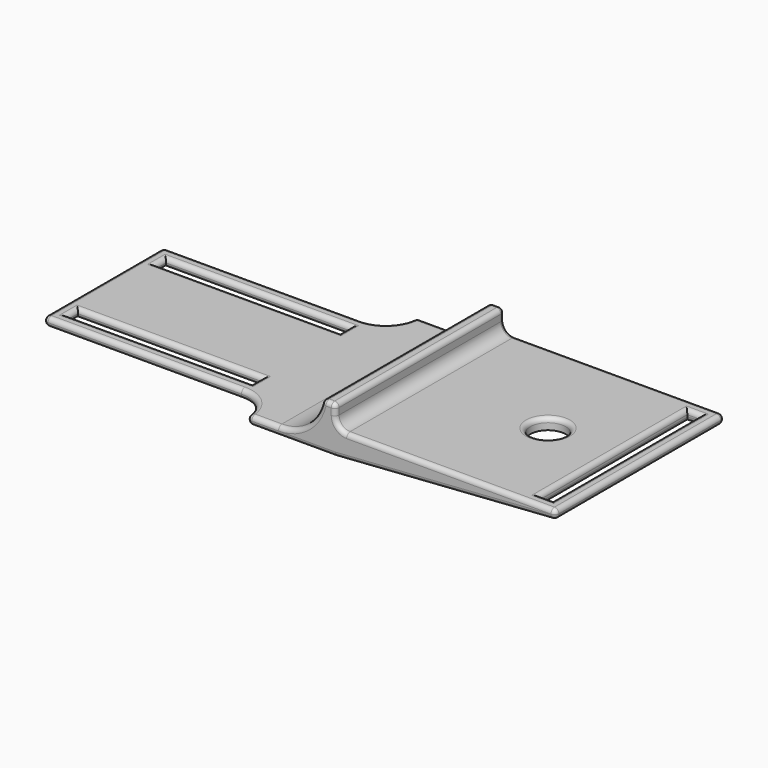
from build123d import *

# Parameters (mm, degrees)
F1_DEPTH = 24
F2_W     = 42
F2_H     = 3
F2_W_2   = 1
F2_H_2   = 6.9865172505
F3_DEPTH = 25
F4_W     = 3
F4_H     = 42
F5_DEPTH = 25
F4_R     = 4
F6_DEPTH = 25
F7_START = -2.5
F4_R_2   = 7.5
F7_DEPTH = 47.5
F8_R     = 0.99999


# Not quite as in the source:
# - a fillet or chamfer is up to 0.001 mm smaller than in the source, because OpenCascade refuses the exact size


with BuildPart() as f1:
    # F0 (on Front) → F1 (new body, symmetric)
    with BuildSketch(Plane.XZ):
        with BuildLine():
            Line((59, 2), (1, 2))
            ThreePointArc((1, 2), (0.2928932188, 1.7071067812), (0, 1))
            ThreePointArc((0, 1), (0.2928932188, 0.2928932188), (1, 0))
            Line((1, 0), (72, 0))
            Line((72, 0), (121.0700975327, 3.4481747867))
            ThreePointArc((121.0700975327, 3.4481747867), (121.7314702772, 3.7638416025), (122, 4.4457149292))
            Line((122, 4.4457149292), (122, 4.5135193938))
            ThreePointArc((122, 4.5135193938), (121.7071067812, 5.220626175), (121, 5.5135193938))
            Line((121, 5.5135193938), (74.5, 5.5135193938))
            ThreePointArc((74.5, 5.5135193938), (72.732233047, 6.2457524408), (72, 8.0135193938))
            Line((72, 8.0135193938), (72, 10.5135193938))
            Line((72, 10.5135193938), (69, 10.5135193938))
            ThreePointArc((69, 10.5135193938), (65.5665823011, 4.4166484237), (59, 2))
        make_face()
    extrude(amount=F1_DEPTH, both=True)

    # F2 (on face) → F3 (cut)
    with BuildSketch(Plane.XY.offset(2)):
        with BuildLine():
            Line((1, 24), (1, 17.0134827495))
            Line((1, 17.0134827495), (45, 17.0134827495))
            ThreePointArc((45, 17.0134827495), (49.9449828941, 19.0589699178), (52, 24))
            Line((52, 24), (1, 24))
        make_face()
        with BuildLine():
            Line((45, -17.0134827495), (1, -17.0134827495))
            Line((1, -17.0134827495), (1, -24))
            Line((1, -24), (52, -24))
            ThreePointArc((52, -24), (49.9449828941, -19.0589699178), (45, -17.0134827495))
        make_face()
        with Locations((24, -12.5134827495)):
            Rectangle(F2_W, F2_H)
        with Locations((24, 12.5134827495)):
            Rectangle(F2_W, F2_H)
        with Locations((0.5, 20.5067413747)):
            Rectangle(F2_W_2, F2_H_2)
        with Locations((0.5, -20.5067413747)):
            Rectangle(F2_W_2, F2_H_2)
    extrude(amount=-F3_DEPTH, mode=Mode.SUBTRACT)

    # F4 (on face) → F5 (cut)
    with BuildSketch(Plane.XY.offset(5.5135193938)):
        with Locations((117.5, 0)):
            Rectangle(F4_W, F4_H)
    extrude(amount=-F5_DEPTH, mode=Mode.SUBTRACT)

    # F4 (on face) → F6 (cut)
    with BuildSketch(Plane.XY.offset(5.5135193938)):
        with Locations((101.1162400246, 0)):
            Circle(F4_R)
    extrude(amount=-F6_DEPTH, mode=Mode.SUBTRACT)

    # F4 (on face) → F7 (cut)
    with BuildSketch(Plane.XY.offset(5.5135193938).offset(F7_START)):
        with Locations((101.1162400246, 0)):
            Circle(F4_R_2)
        with Locations((101.1162400246, 0)):
            Circle(F4_R, mode=Mode.SUBTRACT)
    extrude(amount=-F7_DEPTH, mode=Mode.SUBTRACT)

    # F8 (radius 1 in the source; OpenCascade refuses exactly that, so slightly less here)
    f8_edges = [f1.edges().sort_by_distance(p)[0] for p in [
        (59, 0, 2),
        (55.5, -24, 2),
        (49.944983, -19.05897, 2),
        (23, -17.013483, 2),
        (1, 0, 2),
        (23, 17.013483, 2),
        (49.944983, 19.05897, 2),
        (55.5, 24, 2),
        (3, 12.513483, 2),
        (24, 11.013483, 2),
        (45, 12.513483, 2),
        (24, 14.013483, 2),
        (24, -11.013483, 2),
        (3, -12.513483, 2),
        (24, -14.013483, 2),
        (45, -12.513483, 2),
        (1, 0, 0),
        (23, -17.013483, 0),
        (49.944983, -19.05897, 0),
        (62, -24, 0),
        (72, 0, 0),
        (62, 24, 0),
        (49.944983, 19.05897, 0),
        (23, 17.013483, 0),
        (3, 12.513483, 0),
        (24, 14.013483, 0),
        (45, 12.513483, 0),
        (24, 11.013483, 0),
        (24, -11.013483, 0),
        (45, -12.513483, 0),
        (24, -14.013483, 0),
        (3, -12.513483, 0),
        (121, 0, 5.513519),
        (97.75, 24, 5.513519),
        (97.75, -24, 5.513519),
        (74.5, 0, 5.513519),
        (119, 0, 5.513519),
        (117.5, -21, 5.513519),
        (117.5, 21, 5.513519),
        (116, 0, 5.513519),
        (97.11624, 0, 5.513519),
        (72, 0, 10.513519),
        (69, 0, 10.513519),
        (96.535049, 24, 1.724087),
        (96.535049, -24, 1.724087),
        (121.070098, 0, 3.448175),
        (93.61624, 0, 1.518982),
        (119, 0, 3.302708),
        (117.5, 21, 3.197303),
        (117.5, -21, 3.197303),
        (116, 0, 3.091897),
        (70.5, -24, 10.513519),
        (70.5, 24, 10.513519),
        (52, -24, 1),
        (52, 24, 1),
    ]]
    fillet(f8_edges, radius=F8_R)


solid = f1.part
